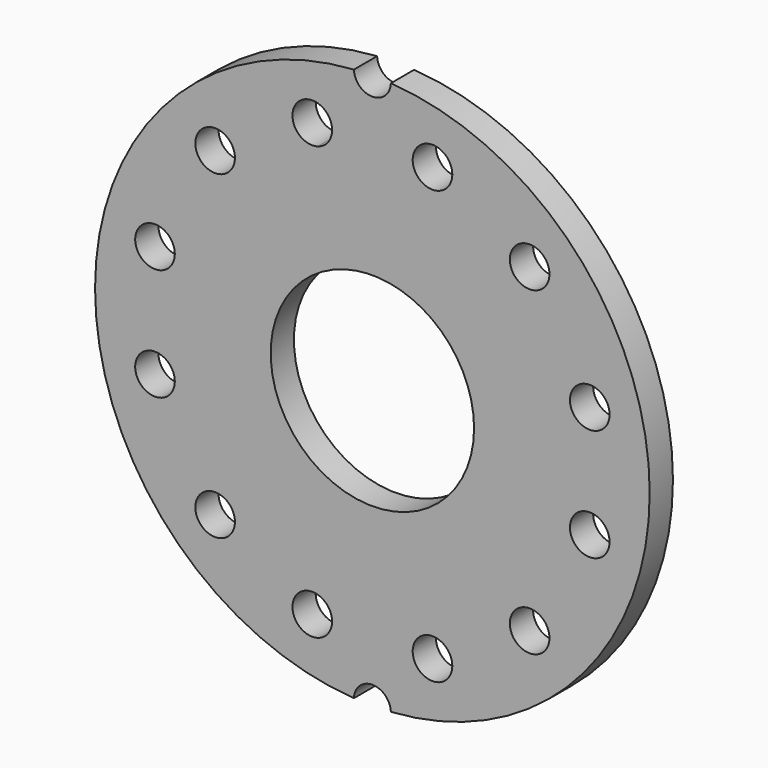
from build123d import *

# Parameters (mm, degrees)
F0_R     = 7.5
F1_DEPTH = 11


# Not quite as in the source:
# - a feature of the source that left no trace in its solid (it failed there, or was rolled back) is left out


with BuildPart() as f1:
    # F0 (on Front) → F1 (new body)
    with BuildSketch(Plane.XZ):
        with BuildLine():
            ThreePointArc((6.9961100303, 104.7666666667), (0, 98), (-6.9961100303, 104.7666666667))
            ThreePointArc((-6.9961100303, 104.7666666667), (-105, 0), (-6.9961100303, -104.7666666667))
            ThreePointArc((-6.9961100303, -104.7666666667), (0, -98), (6.9961100303, -104.7666666667))
            ThreePointArc((6.9961100303, -104.7666666667), (105, 0), (6.9961100303, 104.7666666667))
        make_face()
        with Locations((-59.54553545, -60.6574744609)):
            Circle(F0_R, mode=Mode.SUBTRACT)
        with Locations((-22.7581460876, -81.8966836121)):
            Circle(F0_R, mode=Mode.SUBTRACT)
        with Locations((-82.3036815375, -21.2392091511)):
            Circle(F0_R, mode=Mode.SUBTRACT)
        with Locations((22.7581460876, -81.8966836121)):
            Circle(F0_R, mode=Mode.SUBTRACT)
        with Locations((59.54553545, -60.6574744609)):
            Circle(F0_R, mode=Mode.SUBTRACT)
        with Locations((82.3036815375, -21.2392091511)):
            Circle(F0_R, mode=Mode.SUBTRACT)
        with Locations((-82.3036815375, 21.2392091511)):
            Circle(F0_R, mode=Mode.SUBTRACT)
        with Locations((-59.54553545, 60.6574744609)):
            Circle(F0_R, mode=Mode.SUBTRACT)
        with BuildLine():
            ThreePointArc((-15.2581460876, 81.8966836121), (-16.7869427812, 77.3585418036), (-20.750074374, 74.6705056463))
            ThreePointArc((-20.750074374, 74.6705056463), (-28.729349394, 86.4348254206), (-15.2581460876, 81.8966836121))
        make_face(mode=Mode.SUBTRACT)
        with BuildLine():
            ThreePointArc((10.3081014632, 37.0943802243), (30.6521769727, 23.2957946169), (38.5, 0))
            ThreePointArc((38.5, 0), (-23.2957946169, -30.6521769727), (-10.3081014632, 37.0943802243))
            ThreePointArc((-10.3081014632, 37.0943802243), (0, 38.5), (10.3081014632, 37.0943802243))
        make_face(mode=Mode.SUBTRACT)
        with Locations((82.3036815375, 21.2392091511)):
            Circle(F0_R, mode=Mode.SUBTRACT)
        with BuildLine():
            ThreePointArc((30.2581460876, 81.8966836121), (27.2962878961, 75.9254803057), (20.750074374, 74.6705056463))
            ThreePointArc((20.750074374, 74.6705056463), (18.2200042791, 87.8678869184), (30.2581460876, 81.8966836121))
        make_face(mode=Mode.SUBTRACT)
        with Locations((59.54553545, 60.6574744609)):
            Circle(F0_R, mode=Mode.SUBTRACT)
    extrude(amount=F1_DEPTH)


solid = f1.part
